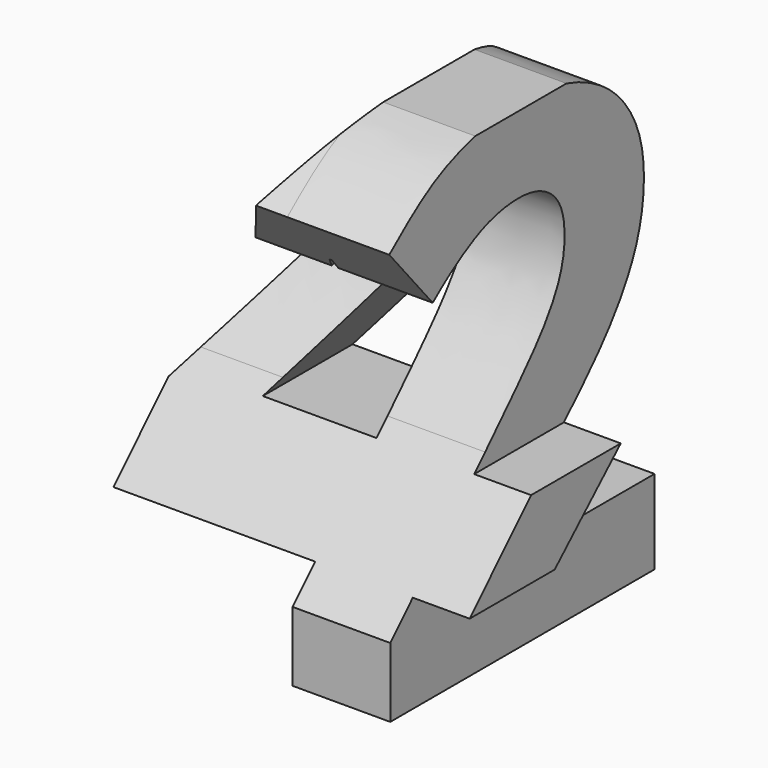
from build123d import *

# Parameters (mm, degrees)
F0_W         = 19.9038460851
F0_H         = 34.4230793417
F2_TEXT_SIZE = 47.5427394526
F3_DEPTH     = 41.7
F4_TEXT_SIZE = 47.5427394526
F5_DEPTH     = 30.9


# Not quite as in the source:
# - Text() gives the source's letters only with a copy of the font that has no kerning and outlines rounded to 1/6400 em; it was checked with that copy


with BuildPart() as f1:
    # F0 (on Front) → F1 (revolve)
    with BuildSketch(Plane.XZ):
        with Locations((9.9519230425, 17.2115396708)):
            Rectangle(F0_W, F0_H)
    revolve(axis=Axis((0, 0, 17.2115396708), (0, 0, -1)))

    # F2 (on Front) → F3 (intersect, symmetric)
    with BuildSketch(Plane.XZ):
        with Locations((-14.9839780707, 0)):
            Text('4', F2_TEXT_SIZE, font='Open Sans', font_style=FontStyle.BOLD, text_align=(TextAlign.LEFT, TextAlign.BOTTOM))
    extrude(amount=F3_DEPTH, both=True, mode=Mode.INTERSECT)

    # F4 (on Right) → F5 (intersect, symmetric)
    with BuildSketch(Plane.YZ):
        with Locations((-14.134616591, 0)):
            Text('2', F4_TEXT_SIZE, font='Open Sans', font_style=FontStyle.BOLD, text_align=(TextAlign.LEFT, TextAlign.BOTTOM))
    extrude(amount=F5_DEPTH, both=True, mode=Mode.INTERSECT)


solid = f1.part
